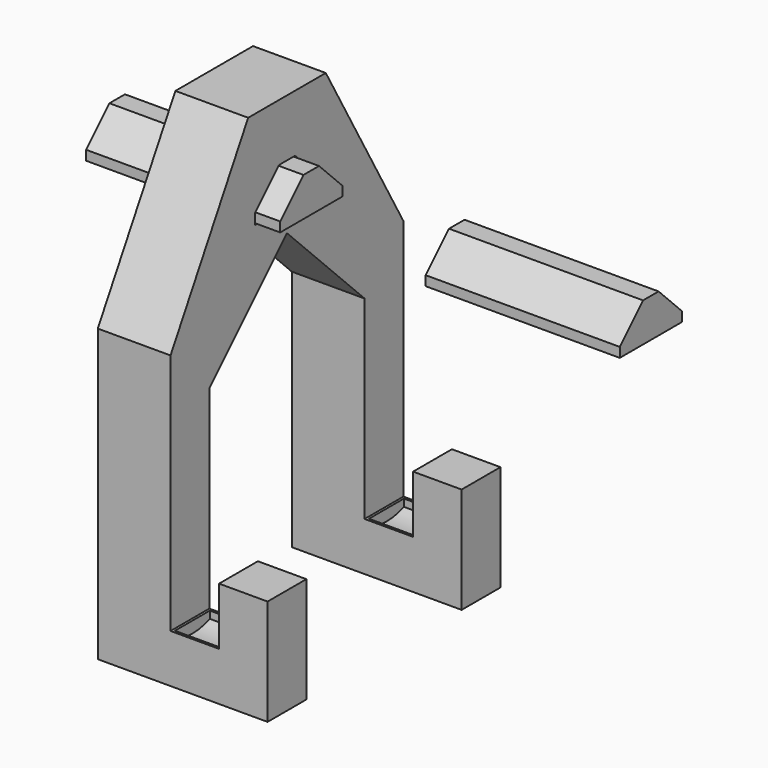
from build123d import *

# Parameters (mm, degrees)
F0_W       = 18
F0_H       = 3
F1_DEPTH   = 60
F2_W       = 80
F2_H       = 100
F3_DEPTH   = 70.001
F6_DEPTH   = 18
F8_DEPTH   = 18
F12_DEPTH  = 40
F13_DEPTH  = 70.001
F14_OFFSET = 0.4


# Not quite as in the source:
# - a pattern or mirror of a feature is missing from the dataset's text; its kind, count and spacing are read off the source's solid


with BuildPart() as f1:
    # F0 (on Front) → F1 (new body, symmetric)
    with BuildSketch(Plane.XZ):
        Polygon((0, 118.4924052926), (0, -71.5075947074), (70, -71.5075947074), (70, -27.8199568838), (50, -27.8199568838), (50, -51.5075947074), (49, -51.5075947074), (49, -54.5075947074), (31, -54.5075947074), (31, -51.5075947074), (30, -51.5075947074), (30, 0), (30, 118.4924052926), align=None)
        with Locations((40, -53.0075947074)):
            Rectangle(F0_W, F0_H)
    extrude(amount=F1_DEPTH, both=True)

    # F2 (on face) → F3 (cut, through all)
    with BuildSketch(Plane(origin=(0, 0, 0), x_dir=(0, -1, 0), z_dir=(-1, 0, 0))):
        with Locations((0, -21.5075947074)):
            Rectangle(F2_W, F2_H)
        Polygon((0, 68.4924052926), (-40, 28.4924052926), (40, 28.4924052926), align=None)
    extrude(amount=-F3_DEPTH, mode=Mode.SUBTRACT)


with BuildPart() as f6:
    # F0 (on Front) → F6 (new body)
    with BuildSketch(Plane.XZ):
        with Locations((40, -53.0075947074)):
            Rectangle(F0_W, F0_H)
    extrude(amount=F6_DEPTH)

    # F7 (on face) → F8 (join, through all)
    with BuildSketch(Plane(origin=(31, 0, 0), x_dir=(0, -1, 0), z_dir=(-1, 0, 0))):
        with BuildLine():
            Line((18, -54.5075947074), (0, -54.5075947074))
            ThreePointArc((0, -54.5075947074), (9, -56.1951463039), (18, -54.5075947074))
        make_face()
    extrude(amount=-F8_DEPTH)


with BuildPart() as f9_1:
    # F9: copy of F6
    add(f6.part.moved(Location((0, -41, 0))))


with BuildPart() as f6_1:
    # F10: moved
    add(f6.part.moved(Location((0, 59, 0))))


with BuildPart() as f1_1:
    add(f1.part)

    # F11: cut F9_1, F6
    add(f9_1.part, mode=Mode.SUBTRACT)
    add(f6_1.part, mode=Mode.SUBTRACT)

    # F5 (on face) → F13 (cut, through all)
    with BuildSketch(Plane(origin=(0, 0, 0), x_dir=(0, -1, 0), z_dir=(-1, 0, 0))):
        Polygon((-20, 118.4924052926), (-40, 118.4924052926), (-40, 98.4924052926), (-31.4285714286, 98.4924052926), align=None)
        Polygon((60, 118.4924052926), (20, 118.4924052926), (60, 48.4924052926), align=None)
    f13 = extrude(amount=-F13_DEPTH, mode=Mode.SUBTRACT)

    # F13_copies: F13 across plane
    add(f13.mirror(Plane.ZX), mode=Mode.SUBTRACT)


with BuildPart() as f12:
    # F5 (on face) → F12 (new body, symmetric)
    with BuildSketch(Plane(origin=(0, 0, 0), x_dir=(0, -1, 0), z_dir=(-1, 0, 0))):
        Polygon((0, 78.4924052926), (0, 94.4924052926), (-4, 94.4924052926), (-16, 82.4924052926), (-16, 78.4924052926), align=None)
        Polygon((4, 94.4924052926), (0, 94.4924052926), (0, 78.4924052926), (16, 78.4924052926), (16, 82.4924052926), align=None)
    extrude(amount=F12_DEPTH, both=True)


with BuildPart() as f1_2:
    add(f1_1.part)

    # F14: cut F12, made larger all round first
    f14_tool = offset(f12.part, amount=F14_OFFSET, kind=Kind.INTERSECTION, mode=Mode.PRIVATE)
    add(f14_tool, mode=Mode.SUBTRACT)


with BuildPart() as f15_1:
    # F15: copy of F12
    add(f12.part.moved(Location((140, 0, 0))))


solid = Compound([f12.part, f1_2.part, f15_1.part])
